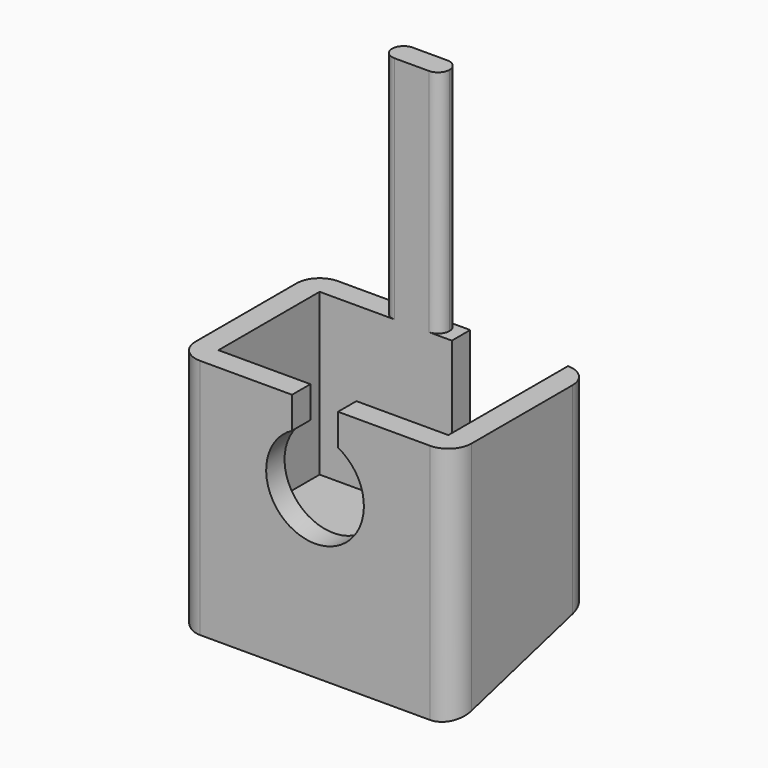
from build123d import *

# Parameters (mm, degrees)
F0_W      = 24
F0_H      = 15
F1_DEPTH  = 16
F2_T      = -2
F4_DEPTH  = 5
F5_W      = 5
F5_H      = 2
F6_DEPTH  = 20
F7_R      = 0.99999
F8_W      = 8.5
F8_H      = 2
F9_DEPTH  = 8
F10_DEPTH = 5
F12_DEPTH = 25
F13_R     = 2
F15_DEPTH = 2


# Not quite as in the source:
# - a fillet or chamfer is up to 0.001 mm smaller than in the source, because OpenCascade refuses the exact size


with BuildPart() as f1:
    # F0 (on Top) → F1 (new body)
    with BuildSketch(Plane.XY):
        Rectangle(F0_W, F0_H)
    extrude(amount=F1_DEPTH)

    # F2
    f2_openings = [f1.faces().sort_by_distance(p)[0] for p in [
        (0, 0, 16),
    ]]
    offset(amount=F2_T, openings=f2_openings)

    # F3 (on face) → F4 (cut)
    with BuildSketch(Plane.XZ.offset(7.5)):
        with BuildLine():
            Line((-2, 16), (-2, 13.25))
            ThreePointArc((-2, 13.25), (0, 5.25), (2, 13.25))
            Line((2, 13.25), (2, 16))
            Line((2, 16), (-2, 16))
        make_face()
    extrude(amount=-F4_DEPTH, mode=Mode.SUBTRACT)

    # F5 (on face) → F6 (join)
    with BuildSketch(Plane.XY.offset(16)):
        with Locations((-2, 6.5)):
            Rectangle(F5_W, F5_H)
    extrude(amount=F6_DEPTH)

    # F7 (radius 1 in the source; OpenCascade refuses exactly that, so slightly less here)
    f7_edges = [f1.edges().sort_by_distance(p)[0] for p in [
        (0.5, 5.5, 26),
        (0.5, 7.5, 26),
        (-4.5, 5.5, 26),
        (-4.5, 7.5, 26),
    ]]
    fillet(f7_edges, radius=F7_R)

    # F8 (on face) → F9 (cut)
    with BuildSketch(Plane.XY.offset(16)):
        with Locations((5.75, 6.5)):
            Rectangle(F8_W, F8_H)
    extrude(amount=-F9_DEPTH, mode=Mode.SUBTRACT)

    # F10 (add): a face of the model
    f10_faces = [f1.faces().sort_by_distance(p)[0] for p in [
        (0, 0, 0),
    ]]
    extrude(f10_faces, amount=F10_DEPTH)

    # F11 (on face) → F12 (cut)
    with BuildSketch(Plane.YZ.offset(12)):
        Polygon((7.5, -0.9807621135), (-7.5, -5), (7.5, -5), align=None)
    extrude(amount=-F12_DEPTH, mode=Mode.SUBTRACT)

    # F13
    f13_edges = [f1.edges().sort_by_distance(p)[0] for p in [
        (12, -7.5, 5.5),
        (-12, -7.5, 5.5),
        (-12, 7.5, 7.509619),
        (12, 7.5, 7.509619),
    ]]
    fillet(f13_edges, radius=F13_R)

    # F14 (on face) → F15 (cut)
    with BuildSketch(Plane(origin=(0, 7.5, 0), x_dir=(-1, 0, 0), z_dir=(0, 1, 0))):
        with BuildLine():
            add(Edge.make_bspline(
                [(-10, 4.0192378865), (-10, 2.0192378865), (-6.5, 2.0192378865), (-3, 2.0192378865), (-3, 4.0192378865)],
                knots=[3.1415926536, 3.1415926536, 3.1415926536, 4.7123889804, 4.7123889804, 6.2831853072, 6.2831853072, 6.2831853072], degree=2, weights=[1, 0.7071067812, 1, 0.7071067812, 1]))
            add(Edge.make_bspline(
                [(-3, 4.0192378865), (-3, 6.0192378865), (-6.5, 6.0192378865), (-10, 6.0192378865), (-10, 4.0192378865)],
                knots=[0, 0, 0, 1.5707963268, 1.5707963268, 3.1415926536, 3.1415926536, 3.1415926536], degree=2, weights=[1, 0.7071067812, 1, 0.7071067812, 1]))
        make_face()
    extrude(amount=-F15_DEPTH, mode=Mode.SUBTRACT)


solid = f1.part
